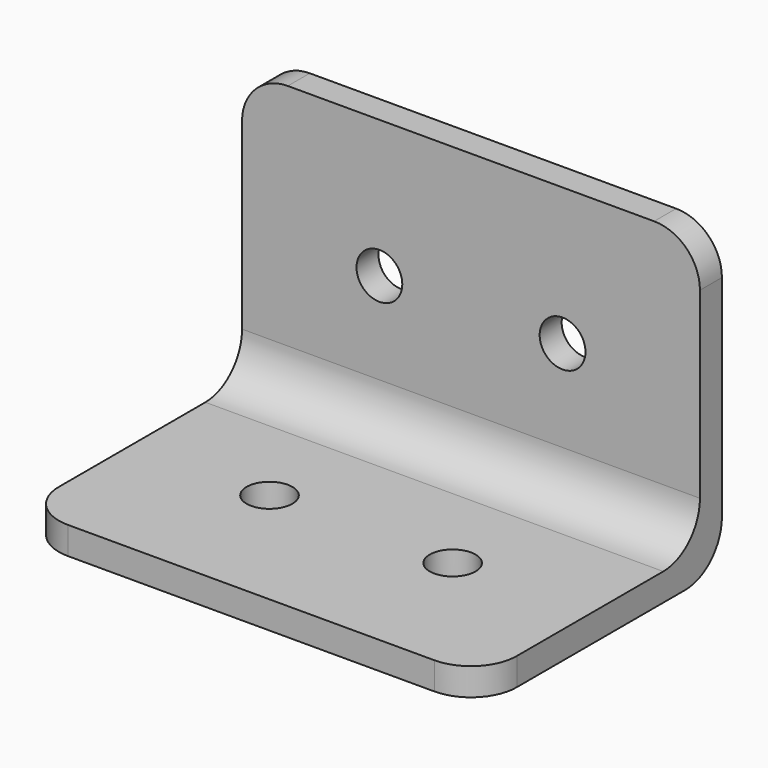
from build123d import *

# Parameters (mm, degrees)
F0_W      = 145
F0_H      = 5
F1_DEPTH  = 360
F0_W_2    = 58
F0_H_2    = 655
F2_DEPTH  = 360
F0_W_3    = 155
F0_H_3    = 163
F0_H_4    = 153
F3_DEPTH  = 360
F5_DEPTH  = 665
F7_DEPTH  = 394
F9_DEPTH  = 125
F11_DEPTH = 50
F12_R     = 5
F14_R     = 2.5
F15_DEPTH = 10
F13_R     = 2.5
F16_DEPTH = 10
F18_DEPTH = 502


# Not quite as in the source:
# - a feature names something its author has since deleted; it is built from what else it names


with BuildPart() as f1:
    # F0 (on Top) → F1 (new body)
    with BuildSketch(Plane.XY):
        Polygon((5, 0), (0, 0), (0, -665), (5, -665), (5, -660), (5, -5), align=None)
        Polygon((155, 0), (5, 0), (5, -5), (150, -5), (155, -5), align=None)
        Polygon((155, -665), (155, -5), (150, -5), (150, -660), (150, -665), align=None)
        with Locations((77.5, -662.5)):
            Rectangle(F0_W, F0_H)
    extrude(amount=-F1_DEPTH)


with BuildPart() as f2:
    # F0 (on Top) → F2 (new body)
    with BuildSketch(Plane.XY):
        Polygon((239, 0), (155, 0), (155, -5), (155, -665), (239, -665), (239, -163), align=None)
        with Locations((197, -332.5)):
            Rectangle(F0_W_2, F0_H_2, mode=Mode.SUBTRACT)
    extrude(amount=-F2_DEPTH)


with BuildPart() as f3:
    # F0 (on Top) → F3 (new body)
    with BuildSketch(Plane.XY):
        with Locations((316.5, -81.5)):
            Rectangle(F0_W_3, F0_H_3)
        with Locations((316.5, -81.5)):
            Rectangle(F0_W, F0_H_4, mode=Mode.SUBTRACT)
    extrude(amount=-F3_DEPTH)


with BuildPart() as f5:
    # F4 (on face) → F5 (new body)
    with BuildSketch(Plane(origin=(0, 0, 0), x_dir=(-1, 0, 0), z_dir=(0, 1, 0))):
        Polygon((0, -330), (0, -360), (30, -360), (30, -359), (1, -359), (1, -330), align=None)
    extrude(amount=-F5_DEPTH)


with BuildPart() as f7:
    # F6 (on face) → F7 (new body)
    with BuildSketch(Plane.YZ.offset(394)):
        Polygon((0, -330), (0, -360), (30, -360), (30, -359), (1, -359), (1, -330), align=None)
    extrude(amount=-F7_DEPTH)


with BuildPart() as f9:
    # F8 (on face) → F9 (new body)
    with BuildSketch(Plane.YZ.offset(394)):
        Polygon((-193, -360), (-163, -360), (-163, -330), (-164, -330), (-164, -359), (-193, -359), align=None)
    extrude(amount=-F9_DEPTH)


with BuildPart() as f11:
    # F10 (on face) → F11 (new body)
    with BuildSketch(Plane.YZ.offset(239)):
        Polygon((-698, -360), (-665, -360), (-665, -327), (-668, -327), (-668, -357), (-698, -357), align=None)
    extrude(amount=-F11_DEPTH)

    # F12
    f12_edges = [f11.edges().sort_by_distance(p)[0] for p in [
        (214, -668, -357),
        (189, -666.5, -327),
        (239, -666.5, -327),
        (239, -698, -358.5),
        (189, -698, -358.5),
        (214, -665, -360),
    ]]
    fillet(f12_edges, radius=F12_R)


with BuildPart() as f15_tool:
    # F14 (on face) → F15 (new body)
    with BuildSketch(Plane.XZ.offset(668)):
        with Locations((204, -342)):
            Circle(F14_R)
        with Locations((224, -342)):
            Circle(F14_R)
    extrude(amount=-F15_DEPTH)


with BuildPart() as f2_1:
    add(f2.part)

    # F15: cut by f15_tool
    add(f15_tool.part, mode=Mode.SUBTRACT)


with BuildPart() as f11_1:
    add(f11.part)

    # F15: cut by f15_tool
    add(f15_tool.part, mode=Mode.SUBTRACT)

    # F13 (on face) → F16 (cut)
    with BuildSketch(Plane.XY.offset(-357)):
        with Locations((204, -683)):
            Circle(F13_R)
        with Locations((224, -683)):
            Circle(F13_R)
    extrude(amount=-F16_DEPTH, mode=Mode.SUBTRACT)


with BuildPart() as f18:
    # F17 (on face) → F18 (new body)
    with BuildSketch(Plane.XZ.offset(665)):
        Polygon((242, -330), (239, -330), (239, -360), (269, -360), (269, -357), (242, -357), align=None)
    extrude(amount=-F18_DEPTH)


solid = f11_1.part
